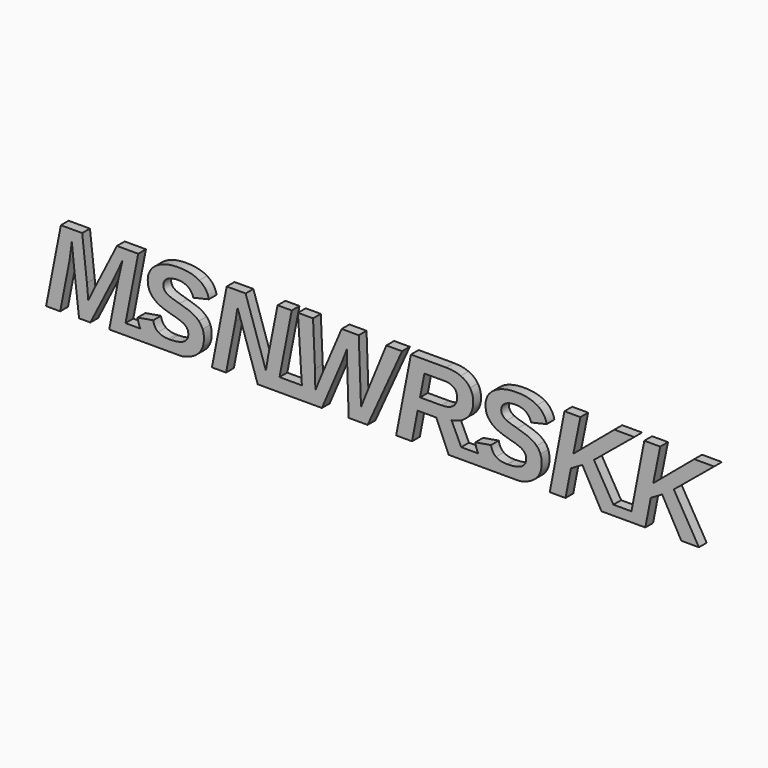
from build123d import *

# Parameters (mm, degrees)
F1_DEPTH = 6.35


# Not quite as in the source:
# - a feature names something its author has since deleted; it is built from what else it names


with BuildPart() as f1:
    # F0 (on Front) → F1 (new body)
    with BuildSketch(Plane.XZ):
        Polygon((-188.0570326252, 7.2882581859), (-188.0570326252, 0.1818913086), (-185.0258379208, 0.1818913086), (-183.6442685256, 7.2882581859), align=None)
        with BuildLine():
            Line((-194.2716674664, 0.1818913086), (-188.0570326252, 0.1818913086))
            Line((-188.0570326252, 0.1818913086), (-188.0570326252, 7.2882581859))
            Line((-188.0570326252, 7.2882581859), (-183.6442685256, 7.2882581859))
            Line((-183.6442685256, 7.2882581859), (-175.3623091162, 49.888103139))
            Line((-175.3623091162, 49.888103139), (-189.2254088499, 49.888103139))
            add(Edge.make_bspline(
                [(-205.5947041382, 17.4656092991), (-204.4996547292, 19.7573106395), (-189.2254088499, 49.888103139)],
                knots=[0, 0, 0, 1, 1, 1], degree=2))
            add(Edge.make_bspline(
                [(-207.9654296627, 12.3516156677), (-206.6897535471, 15.1739079588), (-205.5947041382, 17.4656092991)],
                knots=[0, 0, 0, 1, 1, 1], degree=2))
            Line((-207.9654296627, 12.3516156677), (-208.8459848575, 22.0941686565))
            Line((-208.8459848575, 22.0941686565), (-211.9505063777, 49.888103139))
            Line((-211.9505063777, 49.888103139), (-225.8813411264, 49.888103139))
            Line((-225.8813411264, 49.888103139), (-235.544869931, 0.1818913086))
            Line((-235.544869931, 0.1818913086), (-226.3103295546, 0.1818913086))
            Line((-226.3103295546, 0.1818913086), (-220.2367565442, 31.475468232))
            add(Edge.make_bspline(
                [(-218.7240078762, 42.7307698888), (-219.7061655935, 34.1171338165), (-220.2367565442, 31.475468232)],
                knots=[0, 0, 0, 1, 1, 1], degree=2))
            add(Edge.make_bspline(
                [(-217.3128617307, 29.0708752), (-218.4079111396, 39.3440191395), (-218.7240078762, 42.7307698888)],
                knots=[0, 0, 0, 1, 1, 1], degree=2))
            Line((-217.3128617307, 29.0708752), (-213.9938459964, 0.1818913086))
            Line((-213.9938459964, 0.1818913086), (-206.5881510246, 0.1818913086))
            Line((-206.5881510246, 0.1818913086), (-192.047701141, 28.9692726776))
            add(Edge.make_bspline(
                [(-188.0287569185, 37.4022820433), (-190.8171817021, 31.2609740179), (-192.047701141, 28.9692726776)],
                knots=[0, 0, 0, 1, 1, 1], degree=2))
            Line((-188.0287569185, 37.4022820433), (-185.590296379, 42.7307698888))
            add(Edge.make_bspline(
                [(-188.2093836252, 31.3738657095), (-187.2836717537, 35.9572683902), (-185.590296379, 42.7307698888)],
                knots=[0, 0, 0, 1, 1, 1], degree=2))
            Line((-188.2093836252, 31.3738657095), (-194.2716674664, 0.1818913086))
        make_face()
        with BuildLine():
            Line((-183.6442685256, 7.2882581859), (-185.0258379208, 0.1818913086))
            Line((-185.0258379208, 0.1818913086), (-163.2110848166, 0.1818913086))
            add(Edge.make_bspline(
                [(-163.2110848166, 0.1818913086), (-167.1664679754, 1.0109938063), (-169.8249716411, 2.8066231393)],
                knots=[0.4617336565, 0.4617336565, 0.4617336565, 1, 1, 1], degree=2))
            add(Edge.make_bspline(
                [(-169.8249716411, 2.8066231393), (-172.4136739356, 4.555106632), (-173.9184660336, 7.2882581859)],
                knots=[0, 0, 0, 0.5241336834, 0.5241336834, 0.5241336834], degree=2))
            Line((-173.9184660336, 7.2882581859), (-183.6442685256, 7.2882581859))
        make_face()
        with BuildLine():
            add(Edge.make_bspline(
                [(-163.2110848166, 0.1818913086), (-167.1664679754, 1.0109938063), (-169.8249716411, 2.8066231393)],
                knots=[0.4617336565, 0.4617336565, 0.4617336565, 1, 1, 1], degree=2))
            Line((-163.2110848166, 0.1818913086), (-154.2705546742, 0.1818913086))
            Line((-154.2705546742, 0.1818913086), (-154.2705546742, 7.274382525))
            add(Edge.make_bspline(
                [(-154.7595753914, 7.2714895438), (-154.5125580924, 7.2714895438), (-154.2705546742, 7.274382525)],
                knots=[0, 0, 0, 0.0202976905, 0.0202976905, 0.0202976905], degree=2))
            add(Edge.make_bspline(
                [(-155.691681118, 7.2882581859), (-155.2367460221, 7.2714895438), (-154.7595753914, 7.2714895438)],
                knots=[0.9034977111, 0.9034977111, 0.9034977111, 1, 1, 1], degree=2))
            Line((-155.691681118, 7.2882581859), (-173.9184660336, 7.2882581859))
            add(Edge.make_bspline(
                [(-169.8249716411, 2.8066231393), (-172.4136739356, 4.555106632), (-173.9184660336, 7.2882581859)],
                knots=[0, 0, 0, 0.5241336834, 0.5241336834, 0.5241336834], degree=2))
        make_face()
        with BuildLine():
            Line((-154.2705546742, 7.274382525), (-154.2705546742, 0.1818913086))
            Line((-154.2705546742, 0.1818913086), (-149.5712391788, 0.1818913086))
            Line((-149.5712391788, 0.1818913086), (-146.877915125, 0.1818913086))
            add(Edge.make_bspline(
                [(-138.2548100732, 3.4783287046), (-141.6456599478, 1.1589612566), (-146.877915125, 0.1818913086)],
                knots=[0, 0, 0, 0.5787343015, 0.5787343015, 0.5787343015], degree=2))
            add(Edge.make_bspline(
                [(-132.3957312769, 15.1061729438), (-132.3957312769, 7.4859837579), (-138.2548100732, 3.4783287046)],
                knots=[0, 0, 0, 1, 1, 1], degree=2))
            add(Edge.make_bspline(
                [(-133.2424189642, 20.1524315602), (-132.3957312769, 17.9623327424), (-132.3957312769, 15.1061729438)],
                knots=[0, 0, 0, 1, 1, 1], degree=2))
            add(Edge.make_bspline(
                [(-135.6978132575, 24.0359057528), (-134.0891066516, 22.3425303781), (-133.2424189642, 20.1524315602)],
                knots=[0, 0, 0, 1, 1, 1], degree=2))
            add(Edge.make_bspline(
                [(-139.9876975399, 27.0839814271), (-137.3065198634, 25.7292811274), (-135.6978132575, 24.0359057528)],
                knots=[0, 0, 0, 1, 1, 1], degree=2))
            add(Edge.make_bspline(
                [(-148.2683031219, 29.9965870715), (-142.6688752164, 28.4386817268), (-139.9876975399, 27.0839814271)],
                knots=[0, 0, 0, 1, 1, 1], degree=2))
            add(Edge.make_bspline(
                [(-155.2562988346, 32.2713546581), (-153.495188445, 31.407733217), (-148.2683031219, 29.9965870715)],
                knots=[0, 0, 0, 1, 1, 1], degree=2))
            add(Edge.make_bspline(
                [(-157.9374765111, 34.2977605231), (-157.0174092242, 33.1349760992), (-155.2562988346, 32.2713546581)],
                knots=[0, 0, 0, 1, 1, 1], degree=2))
            add(Edge.make_bspline(
                [(-158.857543798, 37.1200528142), (-158.857543798, 35.460544947), (-157.9374765111, 34.2977605231)],
                knots=[0, 0, 0, 1, 1, 1], degree=2))
            add(Edge.make_bspline(
                [(-156.3513482435, 41.6187867261), (-158.857543798, 39.9762126127), (-158.857543798, 37.1200528142)],
                knots=[0, 0, 0, 1, 1, 1], degree=2))
            add(Edge.make_bspline(
                [(-149.4762442225, 43.2613608395), (-153.8451526891, 43.2613608395), (-156.3513482435, 41.6187867261)],
                knots=[0, 0, 0, 1, 1, 1], degree=2))
            add(Edge.make_bspline(
                [(-142.7196764777, 41.3704250045), (-145.3105408009, 43.2613608395), (-149.4762442225, 43.2613608395)],
                knots=[0, 0, 0, 1, 1, 1], degree=2))
            add(Edge.make_bspline(
                [(-139.3498594821, 36.3072326343), (-140.1288121544, 39.4794891695), (-142.7196764777, 41.3704250045)],
                knots=[0, 0, 0, 1, 1, 1], degree=2))
            Line((-139.3498594821, 36.3072326343), (-129.1896072342, 38.6666689897))
            add(Edge.make_bspline(
                [(-135.4325177821, 47.5794680449), (-130.3523916582, 44.5257477859), (-129.1896072342, 38.6666689897)],
                knots=[0, 0, 0, 1, 1, 1], degree=2))
            add(Edge.make_bspline(
                [(-148.9117857643, 50.6331883038), (-140.512643906, 50.6331883038), (-135.4325177821, 47.5794680449)],
                knots=[0, 0, 0, 1, 1, 1], degree=2))
            add(Edge.make_bspline(
                [(-163.5820610933, 46.8230937109), (-158.0447236182, 50.6331883038), (-148.9117857643, 50.6331883038)],
                knots=[0, 0, 0, 1, 1, 1], degree=2))
            add(Edge.make_bspline(
                [(-169.1193985683, 36.7700885701), (-169.1193985683, 43.0129991179), (-163.5820610933, 46.8230937109)],
                knots=[0, 0, 0, 1, 1, 1], degree=2))
            add(Edge.make_bspline(
                [(-167.4824690395, 30.1546354398), (-169.1193985683, 32.8527468701), (-169.1193985683, 36.7700885701)],
                knots=[0, 0, 0, 1, 1, 1], degree=2))
            add(Edge.make_bspline(
                [(-162.7240842368, 25.5825219283), (-165.8455395107, 27.4565240095), (-167.4824690395, 30.1546354398)],
                knots=[0, 0, 0, 1, 1, 1], degree=2))
            add(Edge.make_bspline(
                [(-153.1113566934, 21.9812769649), (-159.6026289628, 23.708519847), (-162.7240842368, 25.5825219283)],
                knots=[0, 0, 0, 1, 1, 1], degree=2))
            add(Edge.make_bspline(
                [(-144.7065702506, 18.7582191685), (-146.8232894689, 20.4007932819), (-153.1113566934, 21.9812769649)],
                knots=[0, 0, 0, 1, 1, 1], degree=2))
            add(Edge.make_bspline(
                [(-142.5898510323, 14.293352764), (-142.5898510323, 17.115645055), (-144.7065702506, 18.7582191685)],
                knots=[0, 0, 0, 1, 1, 1], degree=2))
            add(Edge.make_bspline(
                [(-154.2705546742, 7.274382525), (-142.5898510323, 7.4140171504), (-142.5898510323, 14.293352764)],
                knots=[0.0202976905, 0.0202976905, 0.0202976905, 1, 1, 1], degree=2))
        make_face()
        with BuildLine():
            add(Edge.make_bspline(
                [(-173.9184660336, 7.2882581859), (-175.2846821263, 9.7697143566), (-175.7574300369, 13.0628333251)],
                knots=[0.5241336834, 0.5241336834, 0.5241336834, 1, 1, 1], degree=2))
            Line((-173.9184660336, 7.2882581859), (-155.691681118, 7.2882581859))
            add(Edge.make_bspline(
                [(-162.261228301, 9.0721120255), (-159.9509875307, 7.4452537347), (-155.691681118, 7.2882581859)],
                knots=[0, 0, 0, 0.9034977111, 0.9034977111, 0.9034977111], degree=2))
            add(Edge.make_bspline(
                [(-165.5633102816, 14.7900762072), (-164.8182251167, 10.8727345072), (-162.261228301, 9.0721120255)],
                knots=[0, 0, 0, 1, 1, 1], degree=2))
            Line((-165.5633102816, 14.7900762072), (-175.7574300369, 13.0628333251))
        make_face()
    extrude(amount=F1_DEPTH)


with BuildPart() as f1b:
    # F0 (on Front) → F1, piece 2 (new body)
    with BuildSketch(Plane.XZ):
        with BuildLine():
            Line((-60.0271709263, 0.1818913086), (-55.3132842231, 0.1818913086))
            add(Edge.make_bspline(
                [(-42.1331792238, 31.1255039879), (-43.2451623865, 28.3370792044), (-55.3132842231, 0.1818913086)],
                knots=[0, 0, 0, 1, 1, 1], degree=2))
            add(Edge.make_bspline(
                [(-38.9101214274, 39.5585133537), (-41.0211960611, 33.9139287715), (-42.1331792238, 31.1255039879)],
                knots=[0, 0, 0, 1, 1, 1], degree=2))
            Line((-38.9101214274, 39.5585133537), (-38.8649647508, 36.5894618634))
            Line((-38.8649647508, 36.5894618634), (-38.7294947208, 28.8338026476))
            Line((-38.7294947208, 28.8338026476), (-37.781204511, 0.1818913086))
            Line((-37.781204511, 0.1818913086), (-25.4308534453, 0.1818913086))
            Line((-25.4308534453, 0.1818913086), (-2.9202501317, 49.888103139))
            Line((-2.9202501317, 49.888103139), (-13.182104902, 49.888103139))
            add(Edge.make_bspline(
                [(-26.9661804516, 16.1447765069), (-25.1486242162, 20.7846250334), (-13.182104902, 49.888103139)],
                knots=[0, 0, 0, 1, 1, 1], degree=2))
            add(Edge.make_bspline(
                [(-29.7320268969, 8.9309974109), (-28.7837366871, 11.5049279804), (-26.9661804516, 16.1447765069)],
                knots=[0, 0, 0, 1, 1, 1], degree=2))
            Line((-29.7320268969, 8.9309974109), (-31.2109080574, 49.888103139))
            Line((-31.2109080574, 49.888103139), (-42.3646071917, 49.888103139))
            Line((-42.3646071917, 49.888103139), (-54.8842957949, 20.5362633118))
            Line((-54.8842957949, 20.5362633118), (-57.571118056, 14.0111235349))
            Line((-57.571118056, 14.0111235349), (-59.5805901672, 8.9309974109))
            add(Edge.make_bspline(
                [(-59.8289518889, 21.1345892775), (-59.5805901672, 15.2077754663), (-59.5805901672, 8.9309974109)],
                knots=[0, 0, 0, 1, 1, 1], degree=2))
            Line((-59.8289518889, 21.1345892775), (-61.0933388353, 49.888103139))
            Line((-61.0933388353, 49.888103139), (-70.971361854, 49.888103139))
            Line((-70.971361854, 49.888103139), (-68.3870872159, 8.9580267668))
            Line((-68.3870872159, 8.9580267668), (-60.0271709263, 8.9580267668))
            Line((-60.0271709263, 8.9580267668), (-60.0271709263, 0.1818913086))
        make_face()
        Polygon((-67.8329728263, 0.1818913086), (-60.0271709263, 0.1818913086), (-60.0271709263, 8.9580267668), (-68.3870872159, 8.9580267668), align=None)
        Polygon((-71.8472877696, 0.1818913086), (-67.8329728263, 0.1818913086), (-68.3870872159, 8.9580267668), (-82.99279761, 8.9580267668), (-84.6989915578, 0.1818913086), align=None)
        Polygon((-91.476008296, 0.1818913086), (-84.6989915578, 0.1818913086), (-82.99279761, 8.9580267668), (-91.476008296, 8.9580267668), align=None)
        with BuildLine():
            Line((-91.476008296, 8.9580267668), (-82.99279761, 8.9580267668))
            Line((-82.99279761, 8.9580267668), (-75.0354627532, 49.888103139))
            Line((-75.0354627532, 49.888103139), (-84.2700031295, 49.888103139))
            Line((-84.2700031295, 49.888103139), (-90.4113111549, 18.6735503997))
            add(Edge.make_bspline(
                [(-91.4386255489, 12.5322423743), (-91.0435046281, 15.4561371879), (-90.4113111549, 18.6735503997)],
                knots=[0, 0, 0, 1, 1, 1], degree=2))
            Line((-91.4386255489, 12.5322423743), (-91.8563248079, 9.6422150683))
            Line((-91.8563248079, 9.6422150683), (-105.1549660835, 49.888103139))
            Line((-105.1549660835, 49.888103139), (-117.5053171492, 49.888103139))
            Line((-117.5053171492, 49.888103139), (-127.1688459538, 0.1818913086))
            Line((-127.1688459538, 0.1818913086), (-117.9343055775, 0.1818913086))
            Line((-117.9343055775, 0.1818913086), (-111.7929975521, 31.6560949387))
            add(Edge.make_bspline(
                [(-110.4495864215, 40.0778151352), (-111.2624066014, 34.3654955381), (-111.7929975521, 31.6560949387)],
                knots=[0, 0, 0, 1, 1, 1], degree=2))
            Line((-110.4495864215, 40.0778151352), (-97.2525476685, 0.1818913086))
            Line((-97.2525476685, 0.1818913086), (-91.476008296, 0.1818913086))
            Line((-91.476008296, 0.1818913086), (-91.476008296, 8.9580267668))
        make_face()
    extrude(amount=F1_DEPTH)


with BuildPart() as f1c:
    # F0 (on Front) → F1, piece 3 (new body)
    with BuildSketch(Plane.XZ):
        Polygon((103.2092291818, 49.888103139), (93.5795678847, 0.1818913086), (103.8752901625, 0.1818913086), (107.4426676184, 18.4251886781), (114.8822300977, 22.7602296372), (127.4019187009, 0.1818913086), (131.4783245325, 0.1818913086), (131.4783245325, 6.5318913086), (135.1821962843, 6.5318913086), (122.5024192836, 28.1564524977), (148.851340113, 49.888103139), (135.8349280666, 49.888103139), (109.0231513014, 27.3436323179), (113.6178431513, 49.888103139), align=None)
        Polygon((131.4783245325, 6.5318913086), (131.4783245325, 0.1818913086), (138.9055820793, 0.1818913086), (135.1821962843, 6.5318913086), align=None)
        Polygon((135.1821962843, 6.5318913086), (138.9055820793, 0.1818913086), (145.758107762, 0.1818913086), (146.9883030834, 6.5318913086), align=None)
        Polygon((146.9883030834, 6.5318913086), (145.758107762, 0.1818913086), (152.4428427219, 0.1818913086), (152.4428427219, 6.5318913086), align=None)
        Polygon((152.4428427219, 6.5318913086), (152.4428427219, 0.1818913086), (156.0538300399, 0.1818913086), (159.6212074958, 18.4251886781), (167.060769975, 22.7602296372), (179.5804585782, 0.1818913086), (191.0841219566, 0.1818913086), (174.6809591609, 28.1564524977), (201.0298799904, 49.888103139), (188.013467944, 49.888103139), (161.2016911788, 27.3436323179), (165.7963830286, 49.888103139), (155.3877690592, 49.888103139), (146.9883030834, 6.5318913086), align=None)
    extrude(amount=F1_DEPTH)


with BuildPart() as f1d:
    # F0 (on Front) → F1, piece 4 (new body)
    with BuildSketch(Plane.XZ):
        with BuildLine():
            Line((72.4347401682, 0.1818913086), (73.8704987135, 0.1818913086))
            add(Edge.make_bspline(
                [(78.5267651081, 1.4506956748), (76.4166605655, 0.6573608995), (73.8704987135, 0.1818913086)],
                knots=[0.2971059881, 0.2971059881, 0.2971059881, 0.5787343015, 0.5787343015, 0.5787343015], degree=2))
            Line((78.5267651081, 1.4506956748), (78.5267651081, 7.2716292925))
            Line((78.5267651081, 7.2716292925), (66.0971784096, 7.2716292925))
            add(Edge.make_bspline(
                [(65.9888384472, 7.2714895438), (66.043129529, 7.2714895438), (66.0971784096, 7.2716292925)],
                knots=[0, 0, 0, 0.0044611595, 0.0044611595, 0.0044611595], degree=2))
            add(Edge.make_bspline(
                [(65.9019015855, 7.2716292925), (65.9452773616, 7.2714895438), (65.9888384472, 7.2714895438)],
                knots=[0.9911902699, 0.9911902699, 0.9911902699, 1, 1, 1], degree=2))
            Line((65.9019015855, 7.2716292925), (46.8391182442, 7.2716292925))
            add(Edge.make_bspline(
                [(50.9234421974, 2.8066231393), (48.3426192445, 4.5497846995), (46.8391182442, 7.2716292925)],
                knots=[0, 0, 0, 0.5225383557, 0.5225383557, 0.5225383557], degree=2))
            add(Edge.make_bspline(
                [(57.5373290219, 0.1818913086), (53.5819458631, 1.0109938063), (50.9234421974, 2.8066231393)],
                knots=[0.4617336565, 0.4617336565, 0.4617336565, 1, 1, 1], degree=2))
            Line((57.5373290219, 0.1818913086), (72.4347401682, 0.1818913086))
        make_face()
        with BuildLine():
            Line((78.5267651081, 7.2716292925), (78.5267651081, 1.4506956748))
            add(Edge.make_bspline(
                [(82.4936037653, 3.4783287046), (80.7528363703, 2.2876303901), (78.5267651081, 1.4506956748)],
                knots=[0, 0, 0, 0.2971059881, 0.2971059881, 0.2971059881], degree=2))
            add(Edge.make_bspline(
                [(88.3526825616, 15.1061729438), (88.3526825616, 7.4859837579), (82.4936037653, 3.4783287046)],
                knots=[0, 0, 0, 1, 1, 1], degree=2))
            add(Edge.make_bspline(
                [(87.5059948743, 20.1524315602), (88.3526825616, 17.9623327424), (88.3526825616, 15.1061729438)],
                knots=[0, 0, 0, 1, 1, 1], degree=2))
            add(Edge.make_bspline(
                [(85.0506005811, 24.0359057528), (86.659307187, 22.3425303781), (87.5059948743, 20.1524315602)],
                knots=[0, 0, 0, 1, 1, 1], degree=2))
            add(Edge.make_bspline(
                [(80.7607162986, 27.0839814271), (83.4418939751, 25.7292811274), (85.0506005811, 24.0359057528)],
                knots=[0, 0, 0, 1, 1, 1], degree=2))
            add(Edge.make_bspline(
                [(72.4801107166, 29.9965870715), (78.0795386221, 28.4386817268), (80.7607162986, 27.0839814271)],
                knots=[0, 0, 0, 1, 1, 1], degree=2))
            add(Edge.make_bspline(
                [(65.4921150039, 32.2713546581), (67.2532253936, 31.407733217), (72.4801107166, 29.9965870715)],
                knots=[0, 0, 0, 1, 1, 1], degree=2))
            add(Edge.make_bspline(
                [(62.8109373274, 34.2977605231), (63.7310046143, 33.1349760992), (65.4921150039, 32.2713546581)],
                knots=[0, 0, 0, 1, 1, 1], degree=2))
            add(Edge.make_bspline(
                [(61.8908700405, 37.1200528142), (61.8908700405, 35.460544947), (62.8109373274, 34.2977605231)],
                knots=[0, 0, 0, 1, 1, 1], degree=2))
            add(Edge.make_bspline(
                [(64.397065595, 41.6187867261), (61.8908700405, 39.9762126127), (61.8908700405, 37.1200528142)],
                knots=[0, 0, 0, 1, 1, 1], degree=2))
            add(Edge.make_bspline(
                [(71.272169616, 43.2613608395), (66.9032611495, 43.2613608395), (64.397065595, 41.6187867261)],
                knots=[0, 0, 0, 1, 1, 1], degree=2))
            add(Edge.make_bspline(
                [(78.0287373609, 41.3704250045), (75.4378730377, 43.2613608395), (71.272169616, 43.2613608395)],
                knots=[0, 0, 0, 1, 1, 1], degree=2))
            add(Edge.make_bspline(
                [(81.3985543564, 36.3072326343), (80.6196016841, 39.4794891695), (78.0287373609, 41.3704250045)],
                knots=[0, 0, 0, 1, 1, 1], degree=2))
            Line((81.3985543564, 36.3072326343), (91.5588066043, 38.6666689897))
            add(Edge.make_bspline(
                [(85.3158960564, 47.5794680449), (90.3960221803, 44.5257477859), (91.5588066043, 38.6666689897)],
                knots=[0, 0, 0, 1, 1, 1], degree=2))
            add(Edge.make_bspline(
                [(71.8366280743, 50.6331883038), (80.2357699325, 50.6331883038), (85.3158960564, 47.5794680449)],
                knots=[0, 0, 0, 1, 1, 1], degree=2))
            add(Edge.make_bspline(
                [(57.1663527453, 46.8230937109), (62.7036902203, 50.6331883038), (71.8366280743, 50.6331883038)],
                knots=[0, 0, 0, 1, 1, 1], degree=2))
            add(Edge.make_bspline(
                [(51.6290152702, 36.7700885701), (51.6290152702, 43.0129991179), (57.1663527453, 46.8230937109)],
                knots=[0, 0, 0, 1, 1, 1], degree=2))
            add(Edge.make_bspline(
                [(53.265944799, 30.1546354398), (51.6290152702, 32.8527468701), (51.6290152702, 36.7700885701)],
                knots=[0, 0, 0, 1, 1, 1], degree=2))
            add(Edge.make_bspline(
                [(58.0243296017, 25.5825219283), (54.9028743278, 27.4565240095), (53.265944799, 30.1546354398)],
                knots=[0, 0, 0, 1, 1, 1], degree=2))
            add(Edge.make_bspline(
                [(67.6370571451, 21.9812769649), (61.1457848757, 23.708519847), (58.0243296017, 25.5825219283)],
                knots=[0, 0, 0, 1, 1, 1], degree=2))
            add(Edge.make_bspline(
                [(76.041843588, 18.7582191685), (73.9251243696, 20.4007932819), (67.6370571451, 21.9812769649)],
                knots=[0, 0, 0, 1, 1, 1], degree=2))
            add(Edge.make_bspline(
                [(78.1585628063, 14.293352764), (78.1585628063, 17.115645055), (76.041843588, 18.7582191685)],
                knots=[0, 0, 0, 1, 1, 1], degree=2))
            add(Edge.make_bspline(
                [(66.0971784096, 7.2716292925), (78.1585628063, 7.3028151958), (78.1585628063, 14.293352764)],
                knots=[0.0044611595, 0.0044611595, 0.0044611595, 1, 1, 1], degree=2))
            Line((66.0971784096, 7.2716292925), (78.5267651081, 7.2716292925))
        make_face()
        with BuildLine():
            Line((39.0641699903, 0.1818913086), (57.5373290219, 0.1818913086))
            add(Edge.make_bspline(
                [(57.5373290219, 0.1818913086), (53.5819458631, 1.0109938063), (50.9234421974, 2.8066231393)],
                knots=[0.4617336565, 0.4617336565, 0.4617336565, 1, 1, 1], degree=2))
            add(Edge.make_bspline(
                [(50.9234421974, 2.8066231393), (48.3426192445, 4.5497846995), (46.8391182442, 7.2716292925)],
                knots=[0, 0, 0, 0.5225383557, 0.5225383557, 0.5225383557], degree=2))
            Line((46.8391182442, 7.2716292925), (35.7333161406, 7.2716292925))
            Line((35.7333161406, 7.2716292925), (39.0641699903, 0.1818913086))
        make_face()
        Polygon((33.7033569813, 0.1818913086), (39.0641699903, 0.1818913086), (35.7333161406, 7.2716292925), (33.7033569813, 7.2716292925), align=None)
        with BuildLine():
            Line((46.8391182442, 7.2716292925), (65.9019015855, 7.2716292925))
            add(Edge.make_bspline(
                [(58.4871855375, 9.0721120255), (61.0216559014, 7.2873525418), (65.9019015855, 7.2716292925)],
                knots=[0, 0, 0, 0.9911902699, 0.9911902699, 0.9911902699], degree=2))
            add(Edge.make_bspline(
                [(55.1851035569, 14.7900762072), (55.9301887218, 10.8727345072), (58.4871855375, 9.0721120255)],
                knots=[0, 0, 0, 1, 1, 1], degree=2))
            Line((55.1851035569, 14.7900762072), (44.9909838016, 13.0628333251))
            add(Edge.make_bspline(
                [(46.8391182442, 7.2716292925), (45.4653165855, 9.7586742734), (44.9909838016, 13.0628333251)],
                knots=[0.5225383557, 0.5225383557, 0.5225383557, 1, 1, 1], degree=2))
        make_face()
        with BuildLine():
            Line((27.5605066119, 0.1818913086), (33.7033569813, 0.1818913086))
            Line((33.7033569813, 0.1818913086), (33.7033569813, 7.2716292925))
            Line((33.7033569813, 7.2716292925), (35.7333161406, 7.2716292925))
            Line((35.7333161406, 7.2716292925), (29.4006411857, 20.7507575259))
            add(Edge.make_bspline(
                [(39.7866768168, 25.7913715578), (35.9596484701, 21.7329152432), (29.4006411857, 20.7507575259)],
                knots=[0, 0, 0, 1, 1, 1], degree=2))
            add(Edge.make_bspline(
                [(43.6137051635, 35.6750391611), (43.6137051635, 29.8498278724), (39.7866768168, 25.7913715578)],
                knots=[0, 0, 0, 1, 1, 1], degree=2))
            add(Edge.make_bspline(
                [(41.5308534527, 43.2218487475), (43.6137051635, 40.0100801202), (43.6137051635, 35.6750391611)],
                knots=[0, 0, 0, 1, 1, 1], degree=2))
            add(Edge.make_bspline(
                [(35.4459912732, 48.1608602568), (39.4480017419, 46.4336173747), (41.5308534527, 43.2218487475)],
                knots=[0, 0, 0, 1, 1, 1], degree=2))
            add(Edge.make_bspline(
                [(25.8332637298, 49.888103139), (31.4439808044, 49.888103139), (35.4459912732, 48.1608602568)],
                knots=[0, 0, 0, 1, 1, 1], degree=2))
            Line((25.8332637298, 49.888103139), (2.8710936496, 49.888103139))
            Line((2.8710936496, 49.888103139), (-6.792435155, 0.1818913086))
            Line((-6.792435155, 0.1818913086), (3.6048896453, 0.1818913086))
            Line((3.6048896453, 0.1818913086), (7.2400021162, 19.0235146438))
            Line((7.2400021162, 19.0235146438), (19.4548831519, 19.0235146438))
            Line((19.4548831519, 19.0235146438), (27.5605066119, 0.1818913086))
        make_face()
        with BuildLine():
            add(Edge.make_bspline(
                [(22.6948747021, 27.1404272729), (27.8088683335, 27.1404272729), (30.4392447488, 29.2007006454)],
                knots=[0, 0, 0, 1, 1, 1], degree=2))
            Line((22.6948747021, 27.1404272729), (8.8317749684, 27.1404272729))
            Line((8.8317749684, 27.1404272729), (11.6879347669, 41.8163471865))
            Line((11.6879347669, 41.8163471865), (24.5350092759, 41.8163471865))
            add(Edge.make_bspline(
                [(30.828721085, 40.0834597198), (28.5878210059, 41.8163471865), (24.5350092759, 41.8163471865)],
                knots=[0, 0, 0, 1, 1, 1], degree=2))
            add(Edge.make_bspline(
                [(33.0696211641, 35.0767131954), (33.0696211641, 38.3505722531), (30.828721085, 40.0834597198)],
                knots=[0, 0, 0, 1, 1, 1], degree=2))
            add(Edge.make_bspline(
                [(30.4392447488, 29.2007006454), (33.0696211641, 31.2609740179), (33.0696211641, 35.0767131954)],
                knots=[0, 0, 0, 1, 1, 1], degree=2))
        make_face(mode=Mode.SUBTRACT)
    extrude(amount=F1_DEPTH)


solid = Compound([f1.part, f1b.part, f1c.part, f1d.part])
